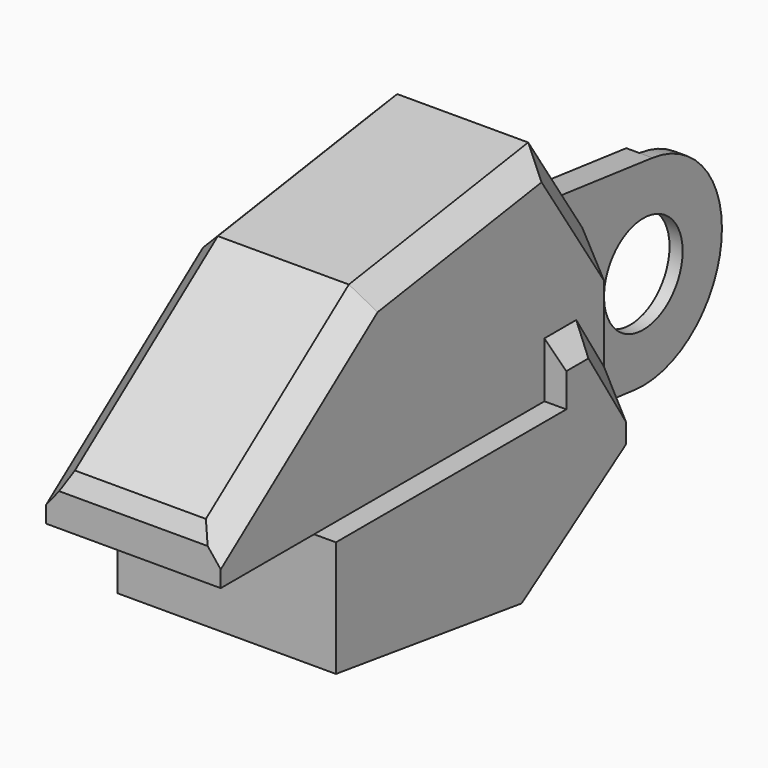
from build123d import *

# Parameters (mm, degrees)
F1_DEPTH      = 20
F1_DEPTH_BACK = 20
F2_DEPTH      = 25
F2_DEPTH_BACK = 25
F3_DEPTH      = 3
F3_DEPTH_BACK = 3
F0_R          = 11.25
F4_DEPTH      = 3
F5_T1_DEPTH   = 79.3350946098
F5_T3_DEPTH   = 53.4182341985
F5_T5_DEPTH   = 77.6393497362
F5_T7_DEPTH   = 53.8076131524
F5_T9_DEPTH   = 40.7011174437
F5_T11_DEPTH  = 34.8143073008


# Not quite as in the source:
# - a fillet or chamfer that OpenCascade refuses, or shapes differently, is made with other operations: its cross-section is extruded or revolved along the edge and cut away or added


with BuildPart() as f1:
    # F0 (on Right) → F1 (new body, two sides)
    with BuildSketch(Plane.YZ) as f1_sk:
        Polygon((0, 0), (0, 26.4743264821), (-15.4693145305, 49.9219790902), (-66.8067783117, 42.1494067516), (-109.735481441, 10.023953287), (-109.735481441, 0), (-83.011649549, 0), (-17.0549713075, 0), (-17.0549713075, 12.6967383549), (-7.9574938864, 12.6967383549), align=None)
    extrude(amount=F1_DEPTH)
    extrude(f1_sk.sketch, amount=-F1_DEPTH_BACK)

    # F0 (on Right) → F2 (join, two sides)
    with BuildSketch(Plane.YZ) as f2_sk:
        Polygon((-29.8482906073, -33.9278131723), (-6.5574786317, -18.399150059), (0, -14.0270879492), (0, 0), (-7.9574938864, 12.6967383549), (-17.0549713075, 12.6967383549), (-17.0549713075, 0), (-83.011649549, 0), (-83.011649549, -26.5361145139), align=None)
    extrude(amount=F2_DEPTH)
    extrude(f2_sk.sketch, amount=-F2_DEPTH_BACK)

    # F0 (on Right) → F3 (join, two sides)
    with BuildSketch(Plane.YZ) as f3_sk:
        with BuildLine():
            ThreePointArc((30.0759126991, -22.3690366524), (10.142147556, 2.5251602116), (35.1261815426, 22.346211547))
            Line((35.1261815426, 22.346211547), (0, 26.4743264821))
            Line((0, 26.4743264821), (0, 0))
            Line((0, 0), (0, -14.0270879492))
            Line((0, -14.0270879492), (-6.5574786317, -18.399150059))
            Line((-6.5574786317, -18.399150059), (30.0759126991, -22.3690366524))
        make_face()
    extrude(amount=F3_DEPTH)
    extrude(f3_sk.sketch, amount=-F3_DEPTH_BACK)

    # F0 (on Right) → F4 (join)
    with BuildSketch(Plane.YZ):
        with BuildLine():
            ThreePointArc((30.0759126991, -22.3690366524), (47.5284403005, -16.7450285797), (55, 0))
            ThreePointArc((55, 0), (49.3127791383, 14.9526070518), (35.1261815426, 22.346211547))
            ThreePointArc((35.1261815426, 22.346211547), (10.142147556, 2.5251602116), (30.0759126991, -22.3690366524))
        make_face()
        with Locations((32.5, 0)):
            Circle(F0_R, mode=Mode.SUBTRACT)
    extrude(amount=F4_DEPTH)

    # F5: chamfer of 5 on 11 edges, made by hand

    # F5_s2 → F5_t1 (cut)
    with BuildSketch(Plane(origin=(0, -12.3102659146, -9.2123182381), x_dir=(1, 0, 0), z_dir=(0, -0.8006358159, -0.5991513084))):
        Polygon((20, 68.7736932965), (15, 73.7736932965), (20, 73.7736932965), align=None)
        Polygon((-20, 68.7736932965), (-15, 73.7736932965), (-20, 73.7736932965), align=None)
    extrude(amount=F5_T1_DEPTH, mode=Mode.SUBTRACT)

    # F5_s4 → F5_t3 (cut)
    with BuildSketch(Plane.YZ.offset(-26.7091170992)):
        Polygon((-107.7312379828, 11.5238176028), (-109.735481441, 7.5206385233), (-109.735481441, 10.023953287), align=None)
    extrude(amount=F5_T3_DEPTH, mode=Mode.SUBTRACT)

    # F5_s6 → F5_t5 (cut)
    with BuildSketch(Plane(origin=(0, 4.9797561094, 0.7539428662), x_dir=(1, 0, 0), z_dir=(0, -0.9887321325, -0.1496955918))):
        Polygon((20, 46.675153037), (15, 51.675153037), (20, 51.675153037), align=None)
        Polygon((-15, 51.675153037), (-20, 46.675153037), (-20, 51.675153037), align=None)
    extrude(amount=F5_T5_DEPTH, mode=Mode.SUBTRACT)

    # F5_s8 → F5_t7 (cut)
    with BuildSketch(Plane(origin=(0, -5.0883568573, 7.7126897705), x_dir=(1, 0, 0), z_dir=(0, -0.5506900388, 0.8347098185))):
        Polygon((15, 14.5791478777), (20, 9.5791478777), (20, 14.5791478777), align=None)
        Polygon((-15, 14.5791478777), (-20, 9.5791478777), (-20, 14.5791478777), align=None)
    extrude(amount=F5_T7_DEPTH, mode=Mode.SUBTRACT)

    # F5_s10 → F5_t9 (cut)
    with BuildSketch(Plane(origin=(0, 6.8285367479, -10.8954082369), x_dir=(1, 0, 0), z_dir=(0, -0.5310558712, 0.8473368053))):
        Polygon((20, 0), (25, -5), (25, 0), align=None)
        Polygon((-25, -5), (-20, 0), (-25, 0), align=None)
    extrude(amount=F5_T9_DEPTH, mode=Mode.SUBTRACT)

    # F5_s12 → F5_t11 (cut)
    with BuildSketch(Plane.XZ.offset(-4.9009210535)):
        Polygon((25, 7.6967383549), (20, 12.6967383549), (25, 12.6967383549), align=None)
        Polygon((-25, 7.6967383549), (-20, 12.6967383549), (-25, 12.6967383549), align=None)
    extrude(amount=F5_T11_DEPTH, mode=Mode.SUBTRACT)


solid = f1.part
